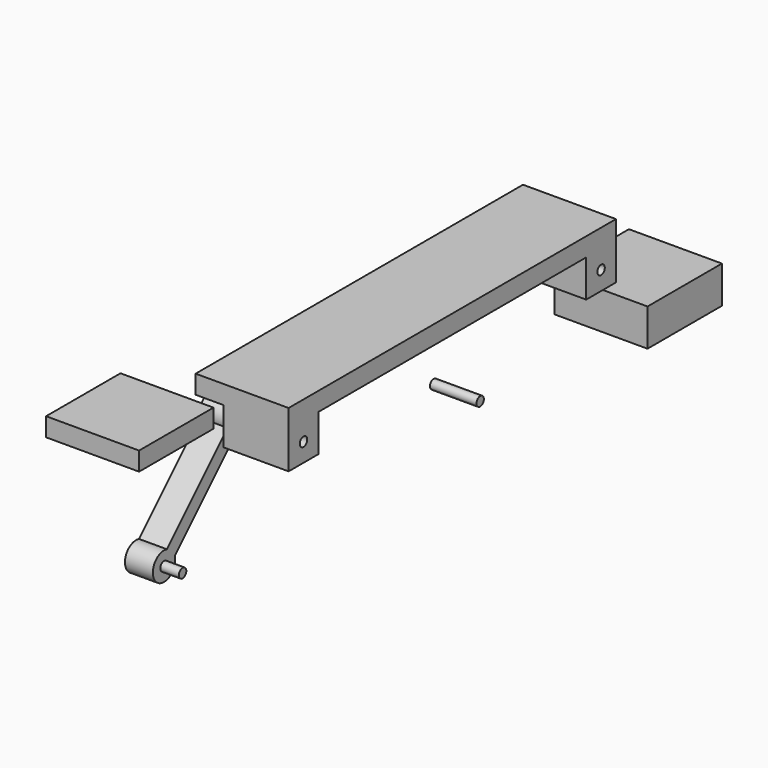
from build123d import *

# Parameters (mm, degrees)
F0_R     = 5
F0_W     = 40
F0_H     = 40
F1_DEPTH = 100
F2_DEPTH = 30
F3_DEPTH = 30
F0_W_2   = 100
F4_DEPTH = 100
F0_H_2   = 20
F5_DEPTH = 100
F6_DEPTH = 50


with BuildPart() as f1:
    # F0 (on Right) → F1 (new body)
    with BuildSketch(Plane.YZ):
        with BuildLine():
            Line((90.6066017178, 80), (120, 80))
            Line((120, 80), (120, 120))
            Line((120, 120), (80, 120))
            Line((80, 120), (80, 90.6066017178))
            Line((80, 90.6066017178), (85.5111126057, 96.1177143235))
            ThreePointArc((85.5111126057, 96.1177143235), (98.0421071167, 114.8716729206), (115, 100))
            ThreePointArc((115, 100), (109.1314214351, 88.0996998956), (96.1177143235, 85.5111126057))
            Line((96.1177143235, 85.5111126057), (90.6066017178, 80))
        make_face()
        with BuildLine():
            Line((80, 80), (90.6066017178, 80))
            Line((90.6066017178, 80), (96.1177143235, 85.5111126057))
            ThreePointArc((96.1177143235, 85.5111126057), (89.3933982822, 89.3933982822), (85.5111126057, 96.1177143235))
            Line((85.5111126057, 96.1177143235), (80, 90.6066017178))
            Line((80, 90.6066017178), (80, 80))
        make_face()
        with BuildLine():
            ThreePointArc((85.5111126057, 96.1177143235), (89.3933982822, 89.3933982822), (96.1177143235, 85.5111126057))
            ThreePointArc((96.1177143235, 85.5111126057), (109.1314214351, 88.0996998956), (115, 100))
            ThreePointArc((115, 100), (98.0421071167, 114.8716729206), (85.5111126057, 96.1177143235))
        make_face()
        with Locations((100, 100)):
            Circle(F0_R, mode=Mode.SUBTRACT)
        Polygon((80, 120), (120, 120), (480, 120), (520, 120), (520, 140), (80, 140), align=None)
        with Locations((500, 100)):
            Rectangle(F0_W, F0_H)
        with Locations((500, 100)):
            Circle(F0_R, mode=Mode.SUBTRACT)
    extrude(amount=F1_DEPTH)

    # F0 (on Right) → F3 (cut)
    with BuildSketch(Plane.YZ):
        with BuildLine():
            Line((90.6066017178, 80), (120, 80))
            Line((120, 80), (120, 120))
            Line((120, 120), (80, 120))
            Line((80, 120), (80, 90.6066017178))
            Line((80, 90.6066017178), (85.5111126057, 96.1177143235))
            ThreePointArc((85.5111126057, 96.1177143235), (98.0421071167, 114.8716729206), (115, 100))
            ThreePointArc((115, 100), (109.1314214351, 88.0996998956), (96.1177143235, 85.5111126057))
            Line((96.1177143235, 85.5111126057), (90.6066017178, 80))
        make_face()
        with BuildLine():
            ThreePointArc((85.5111126057, 96.1177143235), (89.3933982822, 89.3933982822), (96.1177143235, 85.5111126057))
            ThreePointArc((96.1177143235, 85.5111126057), (109.1314214351, 88.0996998956), (115, 100))
            ThreePointArc((115, 100), (98.0421071167, 114.8716729206), (85.5111126057, 96.1177143235))
        make_face()
        with Locations((100, 100)):
            Circle(F0_R, mode=Mode.SUBTRACT)
        with BuildLine():
            Line((80, 80), (90.6066017178, 80))
            Line((90.6066017178, 80), (96.1177143235, 85.5111126057))
            ThreePointArc((96.1177143235, 85.5111126057), (89.3933982822, 89.3933982822), (85.5111126057, 96.1177143235))
            Line((85.5111126057, 96.1177143235), (80, 90.6066017178))
            Line((80, 90.6066017178), (80, 80))
        make_face()
        with Locations((500, 100)):
            Rectangle(F0_W, F0_H)
        with Locations((500, 100)):
            Circle(F0_R, mode=Mode.SUBTRACT)
    extrude(amount=F3_DEPTH, mode=Mode.SUBTRACT)


with BuildPart() as f2:
    # F0 (on Right) → F2 (new body)
    with BuildSketch(Plane.YZ):
        with BuildLine():
            ThreePointArc((85.5111126057, 96.1177143235), (89.3933982822, 89.3933982822), (96.1177143235, 85.5111126057))
            ThreePointArc((96.1177143235, 85.5111126057), (109.1314214351, 88.0996998956), (115, 100))
            ThreePointArc((115, 100), (98.0421071167, 114.8716729206), (85.5111126057, 96.1177143235))
        make_face()
        with Locations((100, 100)):
            Circle(F0_R, mode=Mode.SUBTRACT)
        with BuildLine():
            Line((80, 80), (90.6066017178, 80))
            Line((90.6066017178, 80), (96.1177143235, 85.5111126057))
            ThreePointArc((96.1177143235, 85.5111126057), (89.3933982822, 89.3933982822), (85.5111126057, 96.1177143235))
            Line((85.5111126057, 96.1177143235), (80, 90.6066017178))
            Line((80, 90.6066017178), (80, 80))
        make_face()
        with BuildLine():
            Line((14.4888873943, 3.8822856765), (90.6066017178, 80))
            Line((90.6066017178, 80), (80, 80))
            Line((80, 80), (80, 90.6066017178))
            Line((80, 90.6066017178), (3.8822856765, 14.4888873943))
            ThreePointArc((3.8822856765, 14.4888873943), (10.6066017178, 10.6066017178), (14.4888873943, 3.8822856765))
        make_face()
        with BuildLine():
            ThreePointArc((15, 0), (14.8716729206, 1.9578928833), (14.4888873943, 3.8822856765))
            ThreePointArc((14.4888873943, 3.8822856765), (10.6066017178, 10.6066017178), (3.8822856765, 14.4888873943))
            ThreePointArc((3.8822856765, 14.4888873943), (-11.9003001044, -9.1314214351), (15, 0))
        make_face()
        Circle(F0_R, mode=Mode.SUBTRACT)
    extrude(amount=F2_DEPTH)


with BuildPart() as f4:
    # F0 (on Right) → F4 (new body)
    with BuildSketch(Plane.YZ):
        with Locations((612.4213562373, 20)):
            Rectangle(F0_W_2, F0_H)
    extrude(amount=F4_DEPTH)


with BuildPart() as f5:
    # F0 (on Right) → F5 (new body)
    with BuildSketch(Plane.YZ):
        with Locations((-71, 171.4213562373)):
            Rectangle(F0_W_2, F0_H_2)
    extrude(amount=F5_DEPTH)


with BuildPart() as f6:
    # F0 (on Right) → F6 (new body)
    with BuildSketch(Plane.YZ):
        Circle(F0_R)
    extrude(amount=F6_DEPTH)


with BuildPart() as f6b:
    # F0 (on Right) → F6, piece 2 (new body)
    with BuildSketch(Plane.YZ):
        with Locations((400, 0)):
            Circle(F0_R)
    extrude(amount=F6_DEPTH)


solid = Compound([f1.part, f2.part, f4.part, f5.part, f6.part, f6b.part])
